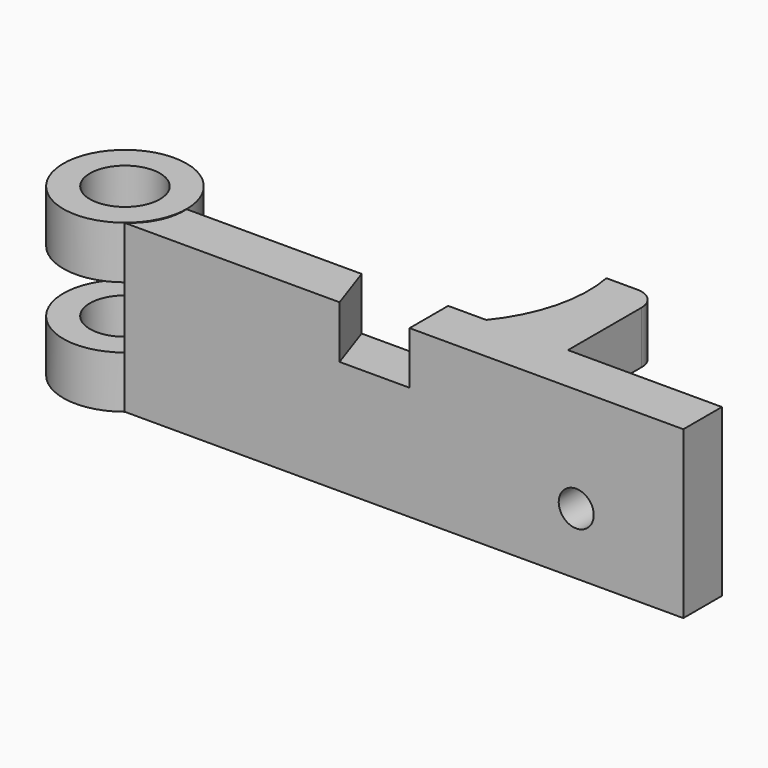
from build123d import *

# Parameters (mm, degrees)
F0_R      = 12.7
F1_DEPTH  = 60.325
F2_DEPTH  = 19.05
F3_R      = 7.874
F4_DEPTH  = 19.05
F5_R      = 6.35
F6_DEPTH  = 22.353
F9_R      = 12.7
F10_DEPTH = 41.402
F8_R      = 12.7
F11_DEPTH = 30.226
F12_DEPTH = 11.176


# Not quite as in the source:
# - a feature names something its author has since deleted; it is built from what else it names


with BuildPart() as f1:
    # F0 (on Top) → F1 (new body)
    with BuildSketch(Plane.XY):
        with BuildLine():
            Line((-10.9417234689, -9.842500207), (66.9919961198, -9.842500207))
            Line((66.9919961198, -9.842500207), (60.9975961198, 7.6517625031))
            Line((60.9975961198, 7.6517625031), (-2.5024038802, 7.6517625031))
            ThreePointArc((-2.5024038802, 7.6517625031), (-4.7224872234, -2.0599745054), (-10.9417234689, -9.842500207))
        make_face()
        Polygon((92.3919961198, 7.6517625031), (92.3919961198, -9.842500207), (191.7059961198, -9.842500207), (191.7059961198, 7.6517625031), (135.8551350103, 7.6517625031), (106.1841961198, 7.6517625031), align=None)
        with BuildLine():
            ThreePointArc((-2.5024038802, 7.6517625031), (-44.986320537, 17.3634995117), (-10.9417234689, -9.842500207))
            ThreePointArc((-10.9417234689, -9.842500207), (-4.7224872234, -2.0599745054), (-2.5024038802, 7.6517625031))
        make_face()
        with Locations((-24.8544038802, 7.6517625031)):
            Circle(F0_R, mode=Mode.SUBTRACT)
        Polygon((60.9975961198, 7.6517625031), (66.9919961198, -9.842500207), (92.3919961198, -9.842500207), (92.3919961198, 7.6517625031), align=None)
    extrude(amount=-F1_DEPTH)

    # F0 (on Top) → F2 (join)
    with BuildSketch(Plane.XY):
        with BuildLine():
            ThreePointArc((116.8051350103, 48.9077037828), (116.0282380438, 27.1126092147), (106.1841961198, 7.6517625031))
            Line((106.1841961198, 7.6517625031), (135.8551350103, 7.6517625031))
            Line((135.8551350103, 7.6517625031), (135.8551350103, 48.9077037828))
            Line((135.8551350103, 48.9077037828), (116.8051350103, 48.9077037828))
        make_face()
    extrude(amount=-F2_DEPTH)

    # F3
    f3_edges = [f1.edges().sort_by_distance(p)[0] for p in [
        (135.855135, 48.907704, -9.525),
    ]]
    fillet(f3_edges, radius=F3_R)

    # F0 (on Top) → F4 (cut)
    with BuildSketch(Plane.XY):
        Polygon((60.9975961198, 7.6517625031), (66.9919961198, -9.842500207), (92.3919961198, -9.842500207), (92.3919961198, 7.6517625031), align=None)
    extrude(amount=-F4_DEPTH, mode=Mode.SUBTRACT)

    # F5 (on face) → F6 (cut, through all)
    with BuildSketch(Plane(origin=(0, 7.6517625031, 0), x_dir=(-1, 0, 0), z_dir=(0, 1, 0))):
        with Locations((-152.8439961198, -37.973)):
            Circle(F5_R)
    extrude(amount=-F6_DEPTH, mode=Mode.SUBTRACT)

    # F9 (on face) → F10 (cut)
    with BuildSketch(Plane.XY):
        with BuildLine():
            ThreePointArc((-2.5024038802, 7.6517625031), (-44.986320537, 17.3634995117), (-10.9417234689, -9.842500207))
            ThreePointArc((-10.9417234689, -9.842500207), (-4.4297129577, -2.2012102715), (-2.5024038802, 7.6517625031))
        make_face()
        with Locations((-24.8544038802, 7.6517625031)):
            Circle(F9_R, mode=Mode.SUBTRACT)
    extrude(amount=-F10_DEPTH, mode=Mode.SUBTRACT)


with BuildPart() as f11:
    # F8 (on offset) → F11 (new body)
    with BuildSketch(Plane.XY.offset(-30.1625)):
        with BuildLine():
            ThreePointArc((-2.5024038802, 7.6517625031), (-44.986320537, 17.3634995117), (-10.9417234689, -9.842500207))
            ThreePointArc((-10.9417234689, -9.842500207), (-4.7224872234, -2.0599745054), (-2.5024038802, 7.6517625031))
        make_face()
        with Locations((-24.8544038802, 7.6517625031)):
            Circle(F8_R, mode=Mode.SUBTRACT)
    extrude(amount=F11_DEPTH)

    # F12 (cut): a face of the model
    f12_faces = [f11.faces().sort_by_distance(p)[0] for p in [
        (-38.373574265, 24.6512127415, -30.1625),
    ]]
    extrude(f12_faces, amount=-F12_DEPTH, mode=Mode.SUBTRACT)


solid = Compound([f1.part, f11.part])
